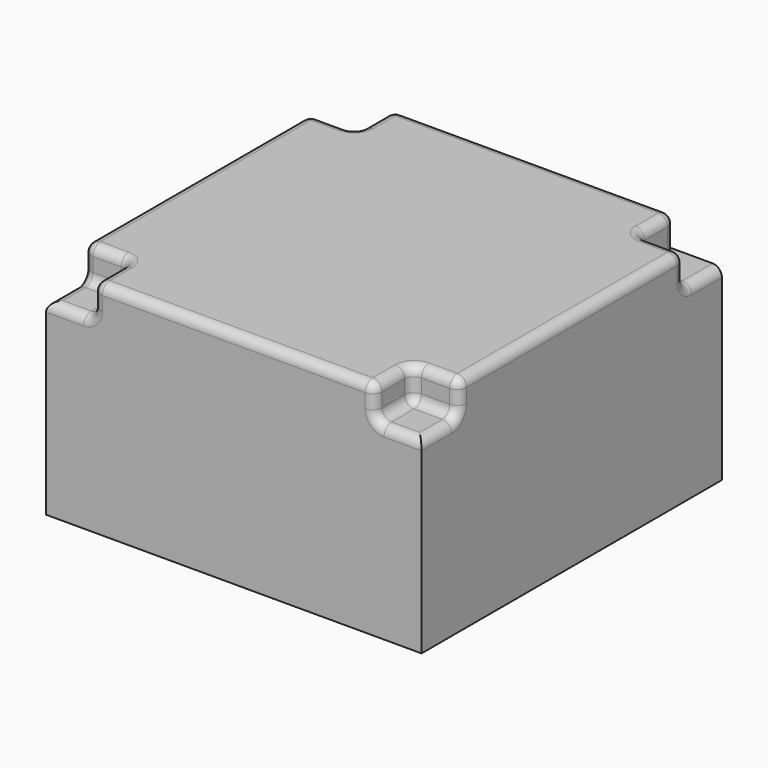
from build123d import *

# Parameters (mm, degrees)
F0_W     = 12.7
F0_H     = 12.7
F1_DEPTH = 50.8
F2_DEPTH = 8.89
F3_F1_R  = 2.54
F3_F2_R  = 2.54


with BuildPart() as f1:
    # F0 (on Top) → F1 (new body)
    with BuildSketch(Plane.XY):
        Polygon((12.7, 12.7), (12.7, 0), (88.9, 0), (88.9, 12.7), (101.6, 12.7), (101.6, 88.9), (88.9, 88.9), (88.9, 101.6), (12.7, 101.6), (12.7, 88.9), (0, 88.9), (0, 12.7), align=None)
        with Locations((6.35, 95.25)):
            Rectangle(F0_W, F0_H)
        with Locations((95.25, 95.25)):
            Rectangle(F0_W, F0_H)
        with Locations((95.25, 6.35)):
            Rectangle(F0_W, F0_H)
        with Locations((6.35, 6.35)):
            Rectangle(F0_W, F0_H)
    extrude(amount=-F1_DEPTH)

    # F0 (on Top) → F2 (join)
    with BuildSketch(Plane.XY):
        Polygon((12.7, 12.7), (12.7, 0), (88.9, 0), (88.9, 12.7), (101.6, 12.7), (101.6, 88.9), (88.9, 88.9), (88.9, 101.6), (12.7, 101.6), (12.7, 88.9), (0, 88.9), (0, 12.7), align=None)
    extrude(amount=F2_DEPTH)

    # F3: fillet of radius 2.54 on 31 edges, made by hand

    # F3_f1
    f3_f1_edges = [f1.edges().sort_by_distance(p)[0] for p in [
        (88.9, 6.35, 0),
        (95.25, 12.7, 0),
        (88.9, 12.7, 4.445),
        (12.7, 12.7, 4.445),
        (6.35, 12.7, 0),
        (12.7, 6.35, 0),
        (12.7, 88.9, 4.445),
        (12.7, 95.25, 0),
        (6.35, 88.9, 0),
        (95.25, 88.9, 0),
        (88.9, 88.9, 4.445),
    ]]
    fillet(f3_f1_edges, radius=F3_F1_R)

    # F3_f2
    f3_f2_edges = [f1.edges().sort_by_distance(p)[0] for p in [
        (50.8, 101.6, 8.89),
        (0, 50.8, 8.89),
        (50.8, 0, 8.89),
        (96.52, 88.9, 8.89),
        (5.08, 88.9, 8.89),
        (5.08, 12.7, 8.89),
        (96.52, 12.7, 8.89),
        (101.6, 50.8, 8.89),
        (88.9, 5.08, 8.89),
        (12.7, 5.08, 8.89),
        (12.7, 96.52, 8.89),
        (88.9, 96.52, 8.89),
        (88.9, 101.6, 4.445),
        (101.6, 12.7, 5.715),
        (88.9, 0, 5.715),
        (12.7, 0, 5.715),
        (0, 12.7, 5.715),
        (0, 88.9, 5.715),
        (12.7, 101.6, 5.715),
        (101.6, 88.9, 5.715),
        (101.6, 89.6439487758, 0.7439487758),
        (11.9560512242, 101.6, 0.7439487758),
        (0, 89.6439487758, 0.7439487758),
        (0, 11.9560512242, 0.7439487758),
        (11.9560512242, 0, 0.7439487758),
        (89.6439487758, 0, 0.7439487758),
        (101.6, 11.9560512242, 0.7439487758),
        (89.6439487758, 89.6439487758, 8.89),
        (11.9560512242, 89.6439487758, 8.89),
        (11.9560512242, 11.9560512242, 8.89),
        (89.6439487758, 11.9560512242, 8.89),
    ]]
    fillet(f3_f2_edges, radius=F3_F2_R)


solid = f1.part
